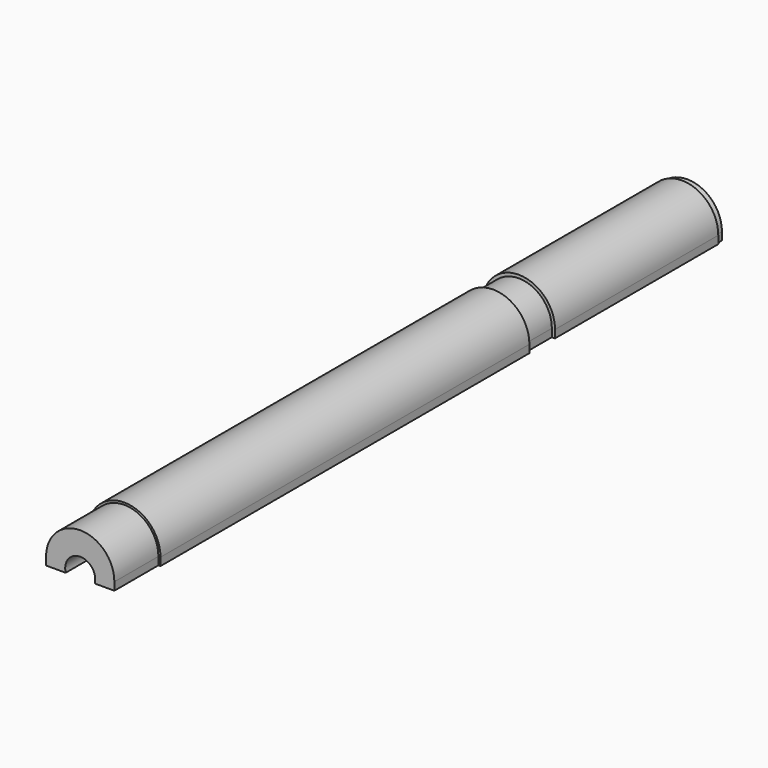
from build123d import *
from build123d import SkipClean  # not in build123d's __all__

# Parameters (mm, degrees)
F1_DEPTH  = 29.21
F3_DEPTH  = 69.05625
F5_DEPTH  = 15.4178
F7_DEPTH  = 6.9596
F9_DEPTH  = 152.4
F11_DEPTH = 89.154
F13_DEPTH = 26.4922
F15_DEPTH = 3.1496


with BuildPart() as f1:
    # F0 (on Front) → F1 (new body)
    with BuildSketch(Plane.XZ):
        with BuildLine():
            Line((11.9332703397, -4.6441399077), (17.4498, -4.6441399077))
            Line((17.4498, -4.6441399077), (17.4498, -0.8595399077))
            ThreePointArc((17.4498, -0.8595399077), (0, 16.6918600923), (-17.4498, -0.8595399077))
            Line((-17.4498, -0.8595399077), (-17.4498, -4.6441399077))
            Line((-17.4498, -4.6441399077), (-11.9332703397, -4.6441399077))
            ThreePointArc((-11.9332703397, -4.6441399077), (0, 9.1988600923), (11.9332703397, -4.6441399077))
        make_face()
    extrude(amount=F1_DEPTH)

    # F2 (on face) → F3 (join)
    with BuildSketch(Plane.XZ.offset(29.21)):
        with BuildLine():
            ThreePointArc((-9.1113708093, -4.6441399077), (0, 6.4977884545), (9.1113708093, -4.6441399077))
            Line((9.1113708093, -4.6441399077), (11.9332703397, -4.6441399077))
            ThreePointArc((11.9332703397, -4.6441399077), (0, 9.1988600923), (-11.9332703397, -4.6441399077))
            Line((-11.9332703397, -4.6441399077), (-9.1113708093, -4.6441399077))
        make_face()
        with BuildLine():
            ThreePointArc((-11.9332703397, -4.6441399077), (0, 9.1988600923), (11.9332703397, -4.6441399077))
            Line((11.9332703397, -4.6441399077), (17.4498, -4.6441399077))
            Line((17.4498, -4.6441399077), (17.4498, -0.8595399077))
            ThreePointArc((17.4498, -0.8595399077), (0, 16.6918600923), (-17.4498, -0.8595399077))
            Line((-17.4498, -0.8595399077), (-17.4498, -4.6441399077))
            Line((-17.4498, -4.6441399077), (-11.9332703397, -4.6441399077))
        make_face()
    extrude(amount=F3_DEPTH)

    # F4 (on face) → F5 (join)
    with BuildSketch(Plane.XZ.offset(98.26625)):
        with BuildLine():
            Line((15.9258256822, -4.6441399077), (15.9258256822, -0.850692377))
            ThreePointArc((15.9258256822, -0.850692377), (0, 15.1678600923), (-15.9258256822, -0.850692377))
            Line((-15.9258256822, -0.850692377), (-15.9038025792, -4.6441399077))
            Line((-15.9038025792, -4.6441399077), (-9.1113708093, -4.6441399077))
            ThreePointArc((-9.1113708093, -4.6441399077), (0, 6.4977884545), (9.1113708093, -4.6441399077))
            Line((9.1113708093, -4.6441399077), (15.9258256822, -4.6441399077))
        make_face()
    extrude(amount=F5_DEPTH)

    # F6 (on face) → F7 (join)
    with BuildSketch(Plane.XZ.offset(113.68405)):
        with BuildLine():
            ThreePointArc((-9.1113708093, -4.6441399077), (0, 6.4977884545), (9.1113708093, -4.6441399077))
            Line((9.1113708093, -4.6441399077), (15.9258256822, -4.6441399077))
            Line((15.9258256822, -4.6441399077), (15.9258256822, -0.850692377))
            ThreePointArc((15.9258256822, -0.850692377), (0, 15.1678600923), (-15.9258256822, -0.850692377))
            Line((-15.9258256822, -0.850692377), (-15.9038025792, -4.6441399077))
            Line((-15.9038025792, -4.6441399077), (-9.1113708093, -4.6441399077))
        make_face()
        with BuildLine():
            Line((15.9258256822, -0.850692377), (15.9258256822, -4.6441399077))
            Line((15.9258256822, -4.6441399077), (17.4498, -4.6441399077))
            Line((17.4498, -4.6441399077), (17.4498, -0.8595399077))
            ThreePointArc((17.4498, -0.8595399077), (0, 16.6918600923), (-17.4498, -0.8595399077))
            Line((-17.4498, -0.8595399077), (-17.4498, -4.6441399077))
            Line((-17.4498, -4.6441399077), (-15.9038025792, -4.6441399077))
            Line((-15.9038025792, -4.6441399077), (-15.9258256822, -0.850692377))
            ThreePointArc((-15.9258256822, -0.850692377), (0, 15.1678600923), (15.9258256822, -0.850692377))
        make_face()
    extrude(amount=F7_DEPTH)

    # F8 (on face) → F9 (join)
    with BuildSketch(Plane.XZ.offset(120.64365)):
        with BuildLine():
            ThreePointArc((17.4498, -0.8595399077), (0, 16.6918600923), (-17.4498, -0.8595399077))
            Line((-17.4498, -0.8595399077), (-17.4498, -4.6441399077))
            Line((-17.4498, -4.6441399077), (-9.1113708093, -4.6441399077))
            ThreePointArc((-9.1113708093, -4.6441399077), (0, 6.4977884545), (9.1113708093, -4.6441399077))
            Line((9.1113708093, -4.6441399077), (17.4498, -4.6441399077))
            Line((17.4498, -4.6441399077), (17.4498, -0.8595399077))
        make_face()
        with BuildLine():
            ThreePointArc((9.1113708093, -4.6441399077), (0, 6.4977884545), (-9.1113708093, -4.6441399077))
            Line((-9.1113708093, -4.6441399077), (-8.4364993371, -4.6441399077))
            ThreePointArc((-8.4364993371, -4.6441399077), (0, 5.8373884545), (8.4364993371, -4.6441399077))
            Line((8.4364993371, -4.6441399077), (9.1113708093, -4.6441399077))
        make_face()
    extrude(amount=F9_DEPTH)

    # F10 (on face) → F11 (join)
    with BuildSketch(Plane.XZ.offset(273.04365)):
        with BuildLine():
            ThreePointArc((17.4498, -0.8595399077), (0, 16.6918600923), (-17.4498, -0.8595399077))
            Line((-17.4498, -0.8595399077), (-17.4498, -4.6441399077))
            Line((-17.4498, -4.6441399077), (-8.4364993371, -4.6441399077))
            ThreePointArc((-8.4364993371, -4.6441399077), (0, 5.8373884545), (8.4364993371, -4.6441399077))
            Line((8.4364993371, -4.6441399077), (17.4498, -4.6441399077))
            Line((17.4498, -4.6441399077), (17.4498, -0.8595399077))
        make_face()
        with BuildLine():
            ThreePointArc((8.4364993371, -4.6441399077), (0, 5.8373884545), (-8.4364993371, -4.6441399077))
            Line((-8.4364993371, -4.6441399077), (-6.9997961445, -4.6441399077))
            ThreePointArc((-6.9997961445, -4.6441399077), (0, 4.4403884545), (6.9997961445, -4.6441399077))
            Line((6.9997961445, -4.6441399077), (8.4364993371, -4.6441399077))
        make_face()
    extrude(amount=F11_DEPTH)

    # F12 (on face) → F13 (cut)
    with BuildSketch(Plane.XZ.offset(362.19765)):
        with BuildLine():
            ThreePointArc((-16.4338, -0.8565464804), (0, 15.6758600923), (16.4338, -0.8565464805))
            Line((16.4338, -0.8565464805), (16.4338, -4.6441399077))
            Line((16.4338, -4.6441399077), (17.4498, -4.6441399077))
            Line((17.4498, -4.6441399077), (17.4498, -0.8595399077))
            ThreePointArc((17.4498, -0.8595399077), (0, 16.6918600923), (-17.4498, -0.8595399077))
            Line((-17.4498, -0.8595399077), (-17.4498, -4.6441399077))
            Line((-17.4498, -4.6441399077), (-16.4338, -4.6441399077))
            Line((-16.4338, -4.6441399077), (-16.4338, -0.8565464804))
        make_face()
    extrude(amount=-F13_DEPTH, mode=Mode.SUBTRACT)

    # F14 (on face) → F15 (join)
    with BuildSketch(Plane(origin=(0, 0, 0), x_dir=(-1, 0, 0), z_dir=(0, 1, 0))):
        with BuildLine():
            ThreePointArc((16.6878128411, -0.8551161423), (0, 15.9298600923), (-16.6878128411, -0.8551161423))
            Line((-16.6878128411, -0.8551161423), (-16.6878128411, -4.6441399077))
            Line((-16.6878128411, -4.6441399077), (-11.9332703397, -4.6441399077))
            ThreePointArc((-11.9332703397, -4.6441399077), (0, 9.1988600923), (11.9332703397, -4.6441399077))
            Line((11.9332703397, -4.6441399077), (16.6658154206, -4.6441399077))
            Line((16.6658154206, -4.6441399077), (16.6878128411, -0.8551161423))
        make_face()
    with SkipClean():  # cleaning this boolean's faces spoils the solid; the shape is the same uncleaned
        extrude(amount=F15_DEPTH)


solid = f1.part
